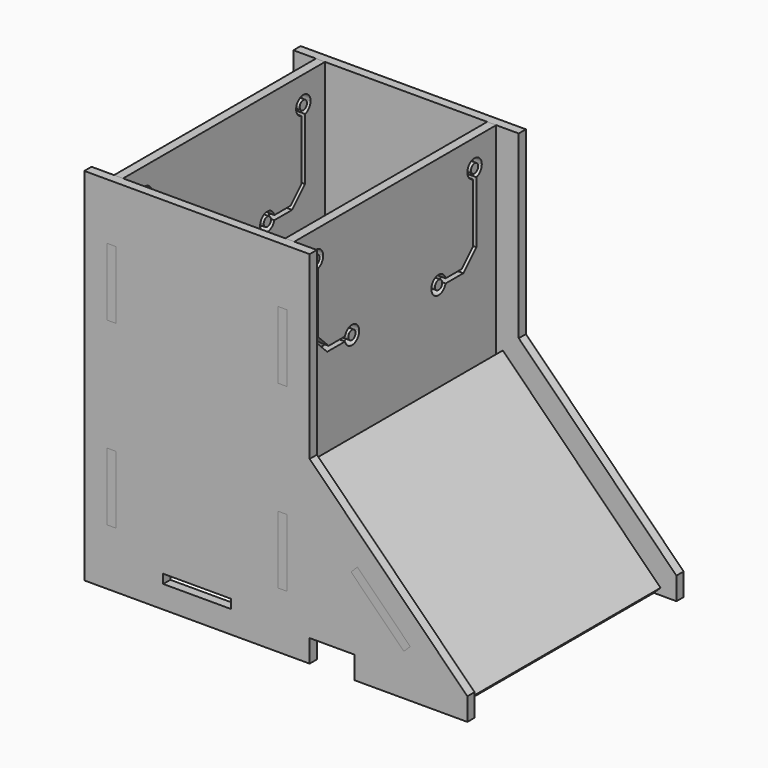
from build123d import *

# Parameters (mm, degrees)
F0_W     = 15
F0_H     = 2
F0_W_2   = 2
F0_H_2   = 15
F1_DEPTH = 30
F2_DEPTH = 28
F3_W     = 15
F3_H     = 2
F3_W_2   = 2
F3_H_2   = 15
F4_DEPTH = 20
F5_DEPTH = 18
F6_W     = 2
F6_H     = 16.5685424949
F7_DEPTH = 2
F9_DEPTH = 40


with BuildPart() as f1:
    # F0 (on Front) → F1 (new body, symmetric)
    with BuildSketch(Plane.XZ):
        Polygon((-25, -40), (25, -40), (25, -35), (25, 0), (25, 40), (-25, 40), align=None)
        with Locations((0, -34)):
            Rectangle(F0_W, F0_H, mode=Mode.SUBTRACT)
        with Locations((-19, -20)):
            Rectangle(F0_W_2, F0_H_2, mode=Mode.SUBTRACT)
        with Locations((19, -20)):
            Rectangle(F0_W_2, F0_H_2, mode=Mode.SUBTRACT)
        with Locations((-19, 20)):
            Rectangle(F0_W_2, F0_H_2, mode=Mode.SUBTRACT)
        with Locations((19, 20)):
            Rectangle(F0_W_2, F0_H_2, mode=Mode.SUBTRACT)
        Polygon((25, 0), (25, -35), (35, -35), (35, -40), (60, -40), (60, -35), align=None)
        Polygon((34.1923881554, -19.091883092), (35.6066017178, -17.6776695297), (47.3223304703, -29.3933982822), (45.908116908, -30.8076118446), align=None, mode=Mode.SUBTRACT)
    extrude(amount=F1_DEPTH, both=True)

    # F0 (on Front) → F2 (cut, symmetric)
    with BuildSketch(Plane.XZ):
        Polygon((-25, -40), (25, -40), (25, -35), (25, 0), (25, 40), (-25, 40), align=None)
        with Locations((0, -34)):
            Rectangle(F0_W, F0_H, mode=Mode.SUBTRACT)
        with Locations((-19, -20)):
            Rectangle(F0_W_2, F0_H_2, mode=Mode.SUBTRACT)
        with Locations((19, -20)):
            Rectangle(F0_W_2, F0_H_2, mode=Mode.SUBTRACT)
        with Locations((-19, 20)):
            Rectangle(F0_W_2, F0_H_2, mode=Mode.SUBTRACT)
        with Locations((19, 20)):
            Rectangle(F0_W_2, F0_H_2, mode=Mode.SUBTRACT)
        Polygon((25, 0), (25, -35), (35, -35), (35, -40), (60, -40), (60, -35), align=None)
        Polygon((34.1923881554, -19.091883092), (35.6066017178, -17.6776695297), (47.3223304703, -29.3933982822), (45.908116908, -30.8076118446), align=None, mode=Mode.SUBTRACT)
    extrude(amount=F2_DEPTH, both=True, mode=Mode.SUBTRACT)


with BuildPart() as f4:
    # F3 (on Right) → F4 (new body, symmetric)
    with BuildSketch(Plane.YZ):
        Polygon((28, -40), (28, -35), (28, -33), (28, -27.5), (28, -12.5), (28, 12.5), (28, 27.5), (28, 40), (-28, 40), (-28, 27.5), (-28, 12.5), (-28, -12.5), (-28, -27.5), (-28, -40), align=None)
        with Locations((0, -34)):
            Rectangle(F3_W, F3_H, mode=Mode.SUBTRACT)
        with Locations((29, 20)):
            Rectangle(F3_W_2, F3_H_2)
        with Locations((-29, 20)):
            Rectangle(F3_W_2, F3_H_2)
        with Locations((29, -20)):
            Rectangle(F3_W_2, F3_H_2)
        with Locations((-29, -20)):
            Rectangle(F3_W_2, F3_H_2)
    extrude(amount=F4_DEPTH, both=True)

    # F3 (on Right) → F5 (cut, symmetric)
    with BuildSketch(Plane.YZ):
        Polygon((28, -40), (28, -35), (28, -33), (28, -27.5), (28, -12.5), (28, 12.5), (28, 27.5), (28, 40), (-28, 40), (-28, 27.5), (-28, 12.5), (-28, -12.5), (-28, -27.5), (-28, -40), align=None)
        with Locations((0, -34)):
            Rectangle(F3_W, F3_H, mode=Mode.SUBTRACT)
        with Locations((29, 20)):
            Rectangle(F3_W_2, F3_H_2)
        with Locations((-29, 20)):
            Rectangle(F3_W_2, F3_H_2)
        with Locations((-29, -20)):
            Rectangle(F3_W_2, F3_H_2)
        with Locations((29, -20)):
            Rectangle(F3_W_2, F3_H_2)
    extrude(amount=F5_DEPTH, both=True, mode=Mode.SUBTRACT)

    # F8 (on face) → F9 (cut, through all)
    with BuildSketch(Plane.YZ.offset(20)):
        with BuildLine():
            ThreePointArc((-21.5, 32.0635083269), (-22, 32), (-22.5, 32.0635083269))
            Line((-22.5, 32.0635083269), (-22.5, 18.8015028834))
            Line((-22.5, 18.8015028834), (-22.5, 18.3872893211))
            Line((-22.5, 18.3872893211), (-18.892569804, 14.7798591251))
            Line((-18.892569804, 14.7798591251), (-18.4783562416, 14.7798591251))
            Line((-18.4783562416, 14.7798591251), (-13.9459307317, 14.7798591251))
            ThreePointArc((-13.9459307317, 14.7798591251), (-14.0094390586, 15.2798591251), (-13.9459307317, 15.7798591251))
            Line((-13.9459307317, 15.7798591251), (-18.4783562416, 15.7798591251))
            Line((-18.4783562416, 15.7798591251), (-21.5, 18.8015028834))
            Line((-21.5, 18.8015028834), (-21.5, 32.0635083269))
        make_face()
        with BuildLine():
            ThreePointArc((-10.0094390586, 15.2798591251), (-11.7574304736, 17.2639185176), (-13.9459307317, 15.7798591251))
            Line((-13.9459307317, 15.7798591251), (-12.8754644624, 15.7798591251))
            ThreePointArc((-12.8754644624, 15.7798591251), (-11.7506200135, 16.2457849514), (-11.0094390586, 15.2798591251))
            ThreePointArc((-11.0094390586, 15.2798591251), (-11.7506200135, 14.3139332988), (-12.8754644624, 14.7798591251))
            Line((-12.8754644624, 14.7798591251), (-13.9459307317, 14.7798591251))
            ThreePointArc((-13.9459307317, 14.7798591251), (-11.7574304736, 13.2957997325), (-10.0094390586, 15.2798591251))
        make_face()
        with BuildLine():
            Line((-12.8754644624, 15.7798591251), (-13.9459307317, 15.7798591251))
            ThreePointArc((-13.9459307317, 15.7798591251), (-14.0094390586, 15.2798591251), (-13.9459307317, 14.7798591251))
            Line((-13.9459307317, 14.7798591251), (-12.8754644624, 14.7798591251))
            ThreePointArc((-12.8754644624, 14.7798591251), (-13.0094390586, 15.2798591251), (-12.8754644624, 15.7798591251))
        make_face()
        with BuildLine():
            ThreePointArc((-21.5, 32.0635083269), (-20.4188611699, 32.7752551286), (-20, 34))
            ThreePointArc((-20, 34), (-23.2247448714, 35.5811388301), (-22.5, 32.0635083269))
            Line((-22.5, 32.0635083269), (-22.5, 33.1339745962))
            ThreePointArc((-22.5, 33.1339745962), (-22.5, 34.8660254038), (-21, 34))
            ThreePointArc((-21, 34), (-21.1339745962, 33.5), (-21.5, 33.1339745962))
            Line((-21.5, 33.1339745962), (-21.5, 32.0635083269))
        make_face()
        with BuildLine():
            Line((-22.5, 33.1339745962), (-22.5, 32.0635083269))
            ThreePointArc((-22.5, 32.0635083269), (-22, 32), (-21.5, 32.0635083269))
            Line((-21.5, 32.0635083269), (-21.5, 33.1339745962))
            ThreePointArc((-21.5, 33.1339745962), (-22, 33), (-22.5, 33.1339745962))
        make_face()
        with BuildLine():
            ThreePointArc((24, 34), (20.7752551286, 35.5811388301), (21.5, 32.0635083269))
            Line((21.5, 32.0635083269), (21.5, 33.1339745962))
            ThreePointArc((21.5, 33.1339745962), (21.5, 34.8660254038), (23, 34))
            ThreePointArc((23, 34), (22.8660254038, 33.5), (22.5, 33.1339745962))
            Line((22.5, 33.1339745962), (22.5, 32.0635083269))
            ThreePointArc((22.5, 32.0635083269), (23.5811388301, 32.7752551286), (24, 34))
        make_face()
        with BuildLine():
            Line((21.5, 33.1339745962), (21.5, 32.0635083269))
            ThreePointArc((21.5, 32.0635083269), (22, 32), (22.5, 32.0635083269))
            Line((22.5, 32.0635083269), (22.5, 33.1339745962))
            ThreePointArc((22.5, 33.1339745962), (22, 33), (21.5, 33.1339745962))
        make_face()
        with BuildLine():
            Line((18.4783562416, 15.7798591251), (13.9459307317, 15.7798591251))
            ThreePointArc((13.9459307317, 15.7798591251), (13.9934984511, 15.53186771), (14.0094390586, 15.2798591251))
            ThreePointArc((14.0094390586, 15.2798591251), (13.9934984511, 15.0278505401), (13.9459307317, 14.7798591251))
            Line((13.9459307317, 14.7798591251), (18.4783562416, 14.7798591251))
            Line((18.4783562416, 14.7798591251), (18.892569804, 14.7798591251))
            Line((18.892569804, 14.7798591251), (22.5, 18.3872893211))
            Line((22.5, 18.3872893211), (22.5, 18.8015028834))
            Line((22.5, 18.8015028834), (22.5, 32.0635083269))
            ThreePointArc((22.5, 32.0635083269), (22, 32), (21.5, 32.0635083269))
            Line((21.5, 32.0635083269), (21.5, 18.8015028834))
            Line((21.5, 18.8015028834), (18.4783562416, 15.7798591251))
        make_face()
        with BuildLine():
            ThreePointArc((12.8754644624, 15.7798591251), (12.9753648849, 15.5386781702), (13.0094390586, 15.2798591251))
            ThreePointArc((13.0094390586, 15.2798591251), (12.9753648849, 15.02104008), (12.8754644624, 14.7798591251))
            Line((12.8754644624, 14.7798591251), (13.9459307317, 14.7798591251))
            ThreePointArc((13.9459307317, 14.7798591251), (13.9934984511, 15.0278505401), (14.0094390586, 15.2798591251))
            ThreePointArc((14.0094390586, 15.2798591251), (13.9934984511, 15.53186771), (13.9459307317, 15.7798591251))
            Line((13.9459307317, 15.7798591251), (12.8754644624, 15.7798591251))
        make_face()
        with BuildLine():
            ThreePointArc((12.8754644624, 14.7798591251), (11.0094390586, 15.2798591251), (12.8754644624, 15.7798591251))
            Line((12.8754644624, 15.7798591251), (13.9459307317, 15.7798591251))
            ThreePointArc((13.9459307317, 15.7798591251), (10.0094390586, 15.2798591251), (13.9459307317, 14.7798591251))
            Line((13.9459307317, 14.7798591251), (12.8754644624, 14.7798591251))
        make_face()
    extrude(amount=-F9_DEPTH, mode=Mode.SUBTRACT)


with BuildPart() as f7:
    # F6 (on face) → F7 (new body)
    with BuildSketch(Plane(origin=(7.5502525317, 0, 7.5502525317), x_dir=(0, 1, 0), z_dir=(0.7071067812, 0, 0.7071067812))):
        with Locations((-29, -45.9619407771)):
            Rectangle(F6_W, F6_H)
        Polygon((28, -17.6776695297), (-28, -17.6776695297), (-28, -37.6776695297), (-28, -54.2462120246), (-28, -67.1751442127), (28, -67.1751442127), (28, -54.2462120246), (28, -37.6776695297), align=None)
        with Locations((29, -45.9619407771)):
            Rectangle(F6_W, F6_H)
    extrude(amount=F7_DEPTH)


solid = Compound([f1.part, f4.part, f7.part])
